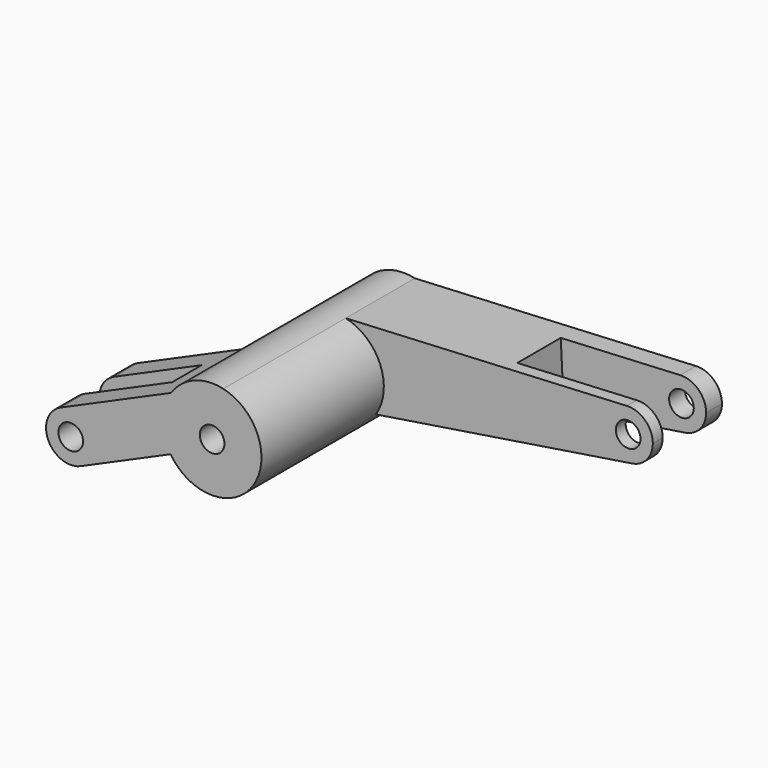
from build123d import *

# Parameters (mm, degrees)
F0_R     = 5
F1_DEPTH = 97
F2_DEPTH = 35
F3_R     = 5
F4_DEPTH = 58
F5_W     = 21.1601814699
F5_H     = 15
F5_W_2   = 38.8398185301
F6_DEPTH = 94.4868054059
F7_W     = 48.4832398096
F7_H     = 22
F7_W_2   = 11.5167601904
F8_DEPTH = 53.4786196206


with BuildPart() as f1:
    # F0 (on Front) → F1 (new body)
    with BuildSketch(Plane.XZ):
        with BuildLine():
            Line((-33.3940822773, -3.829139489), (-78.1385323231, -23.6095790069))
            ThreePointArc((-78.1385323231, -23.6095790069), (-83.2413837038, -36.7990030954), (-70.0519596153, -41.9018544761))
            Line((-70.0519596153, -41.9018544761), (-33.6129821019, -25.7930635521))
            ThreePointArc((-33.6129821019, -25.7930635521), (-16.8207912618, -34.9776541604), (0, -25.8455482049))
            ThreePointArc((0, -25.8455482049), (1.7560740266, -7.4903982751), (-12.2514262399, 4.5006509372))
            ThreePointArc((-12.2514262399, 4.5006509372), (-24.1207121326, 3.6302295915), (-33.3940822773, -3.829139489))
        make_face()
        with Locations((-74.0952459692, -32.7557167415)):
            Circle(F0_R, mode=Mode.SUBTRACT)
        with Locations((-16.789562501, -14.9776785413)):
            Circle(F0_R, mode=Mode.SUBTRACT)
    extrude(amount=F1_DEPTH)

    # F0 (on Front) → F2 (join)
    with BuildSketch(Plane.XZ):
        with BuildLine():
            Line((-33.3940822773, -3.829139489), (-78.1385323231, -23.6095790069))
            ThreePointArc((-78.1385323231, -23.6095790069), (-83.2413837038, -36.7990030954), (-70.0519596153, -41.9018544761))
            Line((-70.0519596153, -41.9018544761), (-33.6129821019, -25.7930635521))
            ThreePointArc((-33.6129821019, -25.7930635521), (-16.8207912618, -34.9776541604), (0, -25.8455482049))
            ThreePointArc((0, -25.8455482049), (1.7560740266, -7.4903982751), (-12.2514262399, 4.5006509372))
            ThreePointArc((-12.2514262399, 4.5006509372), (-24.1207121326, 3.6302295915), (-33.3940822773, -3.829139489))
        make_face()
        with Locations((-74.0952459692, -32.7557167415)):
            Circle(F0_R, mode=Mode.SUBTRACT)
        with Locations((-16.789562501, -14.9776785413)):
            Circle(F0_R, mode=Mode.SUBTRACT)
        with BuildLine():
            Line((101.7329280454, 10.2593952934), (-12.2514262399, 4.5006509372))
            ThreePointArc((-12.2514262399, 4.5006509372), (1.7560740266, -7.4903982751), (0, -25.8455482049))
            Line((0, -25.8455482049), (103.7832955951, -9.6076711141))
            ThreePointArc((103.7832955951, -9.6076711141), (92.2903408389, -0.7544573444), (101.7329280454, 10.2593952934))
        make_face()
        with BuildLine():
            ThreePointArc((112.2375068401, 0.2721333944), (109.1278701125, 7.5194014295), (101.7329280454, 10.2593952934))
            ThreePointArc((101.7329280454, 10.2593952934), (92.2903408389, -0.7544573444), (103.7832955951, -9.6076711141))
            ThreePointArc((103.7832955951, -9.6076711141), (109.8354633926, -6.2294861135), (112.2375068401, 0.2721333944))
        make_face()
        with Locations((102.2375068401, 0.2721333944)):
            Circle(F0_R, mode=Mode.SUBTRACT)
    extrude(amount=F2_DEPTH)

    # F3 (on face) → F4 (cut)
    with BuildSketch(Plane(origin=(0, 0, 0), x_dir=(-1, 0, 0), z_dir=(0, 1, 0))):
        with BuildLine():
            ThreePointArc((33.3940822773, -3.829139489), (31.8014961432, -14.0586725369), (25.3075095695, -22.1214149583))
            Line((25.3075095695, -22.1214149583), (33.6129821019, -25.7930635521))
            Line((33.6129821019, -25.7930635521), (70.0519596153, -41.9018544761))
            ThreePointArc((70.0519596153, -41.9018544761), (64.9491082346, -28.7124303876), (78.1385323231, -23.6095790069))
            Line((78.1385323231, -23.6095790069), (33.3940822773, -3.829139489))
        make_face()
        with BuildLine():
            ThreePointArc((84.0952459692, -32.7557167415), (82.4747705243, -27.2982843571), (78.1385323231, -23.6095790069))
            ThreePointArc((78.1385323231, -23.6095790069), (64.9491082346, -28.7124303876), (70.0519596153, -41.9018544761))
            ThreePointArc((70.0519596153, -41.9018544761), (79.5526783536, -41.1352412966), (84.0952459692, -32.7557167415))
        make_face()
        with Locations((74.0952459692, -32.7557167415)):
            Circle(F3_R, mode=Mode.SUBTRACT)
    extrude(amount=-F4_DEPTH, mode=Mode.SUBTRACT)

    # F5 (on face) → F6 (cut, through all)
    with BuildSketch(Plane(origin=(-4.0432863539, 0, 9.1461377346), x_dir=(0.9146137735, 0, 0.4043286354), z_dir=(-0.4043286354, 0, 0.9146137735))):
        with Locations((-91.5926974976, -77.5)):
            Rectangle(F5_W, F5_H)
        with Locations((-61.5926974976, -77.5)):
            Rectangle(F5_W_2, F5_H)
    extrude(amount=-F6_DEPTH, mode=Mode.SUBTRACT)

    # F7 (on face) → F8 (cut, through all)
    with BuildSketch(Plane(origin=(-0.2579961306, 0, 5.1065858341), x_dir=(0.9987261899, 0, 0.0504578795), z_dir=(-0.0504578795, 0, 0.9987261899))):
        with Locations((77.8793870409, -19)):
            Rectangle(F7_W, F7_H)
        with Locations((107.8793870409, -19)):
            Rectangle(F7_W_2, F7_H)
    extrude(amount=-F8_DEPTH, mode=Mode.SUBTRACT)


solid = f1.part
